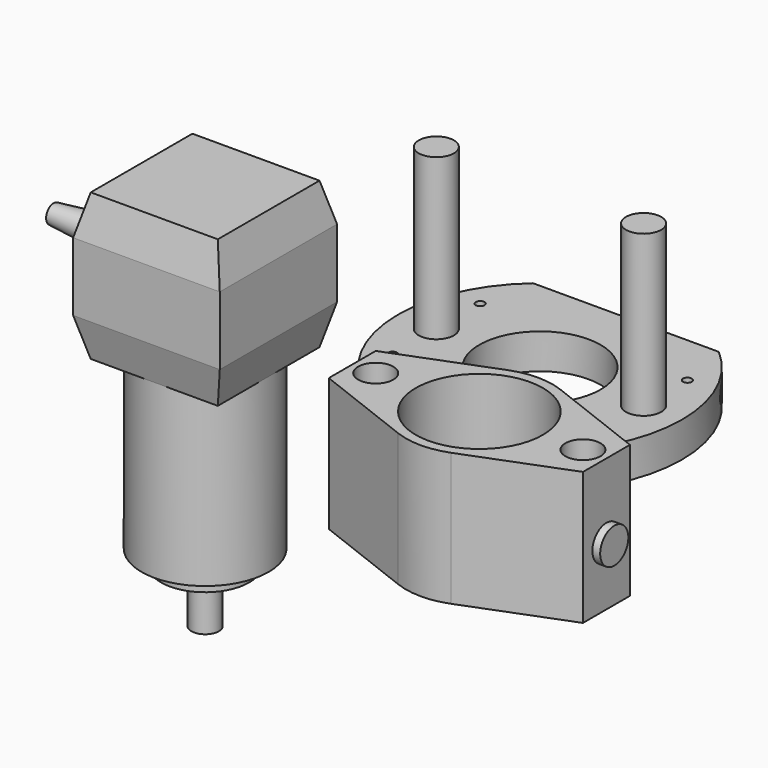
from build123d import *

# Parameters (mm, degrees)
F0_R         = 9
F0_R_2       = 31
F1_DEPTH     = 18
F2_DEPTH     = 100
F3_R         = 4.5
F4_DEPTH     = 100
F5_R         = 9
F5_R_2       = 32.5
F6_DEPTH     = 68
F7_R         = 9
F8_DEPTH     = 4
F9_R         = 9
F10_DEPTH    = 4
F16_W        = 75
F16_H        = 75
F17_DEPTH    = 75
F18_SIZE2    = 5
F18_SIZE     = 20
F19_C1_SIZE2 = 5
F19_C1_SIZE  = 20
F19_C2_SIZE2 = 5
F19_C2_SIZE  = 20
F19_C3_SIZE2 = 5
F19_C3_SIZE  = 20
F19_C4_SIZE2 = 20
F19_C4_SIZE  = 5
F19_C5_SIZE2 = 20
F19_C5_SIZE  = 5
F19_C6_SIZE2 = 5
F19_C6_SIZE  = 20
F19_C7_SIZE2 = 5
F19_C7_SIZE  = 20
F20_R        = 9
F21_DEPTH    = 40
F21_TAPER    = 6
F22_R        = 32.5
F23_DEPTH    = 88
F24_R        = 22.5
F25_DEPTH    = 8
F26_R        = 7
F27_DEPTH    = 27
F28_R        = 2.25
F29_DEPTH    = 25


# Not quite as in the source:
# - a feature of the source that left no trace in its solid (it failed there, or was rolled back) is left out


with BuildPart() as f1:
    # F0 (on Top) → F1 (new body)
    with BuildSketch(Plane.XY):
        with BuildLine():
            Line((47.5, 55), (-47.5, 55))
            ThreePointArc((-47.5, 55), (-72.6722092687, 0), (-47.5, -55))
            Line((-47.5, -55), (47.5, -55))
            ThreePointArc((47.5, -55), (72.6722092687, 0), (47.5, 55))
        make_face()
        with Locations((-53, 0)):
            Circle(F0_R, mode=Mode.SUBTRACT)
        Circle(F0_R_2, mode=Mode.SUBTRACT)
        with Locations((53, 0)):
            Circle(F0_R, mode=Mode.SUBTRACT)
    extrude(amount=F1_DEPTH)

    # F0 (on Top) → F2 (join)
    with BuildSketch(Plane.XY):
        with Locations((-53, 0)):
            Circle(F0_R)
        with Locations((53, 0)):
            Circle(F0_R)
    extrude(amount=F2_DEPTH)

    # F3 (on Right) → F4 (cut, symmetric)
    with BuildSketch(Plane.YZ):
        with Locations((-41.5, 9)):
            Circle(F3_R)
        with Locations((41.5, 9)):
            Circle(F3_R)
    extrude(amount=F4_DEPTH, both=True, mode=Mode.SUBTRACT)

    # F28 (on face) → F29 (cut)
    with BuildSketch(Plane.XY):
        with Locations((-53, 28)):
            Circle(F28_R)
        with Locations((-53, -28)):
            Circle(F28_R)
        with Locations((53, -28)):
            Circle(F28_R)
        with Locations((53, 28)):
            Circle(F28_R)
    extrude(amount=F29_DEPTH, mode=Mode.SUBTRACT)


with BuildPart() as f6:
    # F5 (on Top) → F6 (new body)
    with BuildSketch(Plane.XY):
        with BuildLine():
            Line((0, -105), (0, -135))
            Line((0, -135), (51.4330297899, -154.9597957562))
            ThreePointArc((51.4330297899, -154.9597957562), (65, -157.5), (78.5669702101, -154.9597957562))
            Line((78.5669702101, -154.9597957562), (130, -135))
            Line((130, -135), (130, -105))
            Line((130, -105), (78.5669702101, -85.0402042438))
            ThreePointArc((78.5669702101, -85.0402042438), (65, -82.5), (51.4330297899, -85.0402042438))
            Line((51.4330297899, -85.0402042438), (0, -105))
        make_face()
        with Locations((12, -120)):
            Circle(F5_R, mode=Mode.SUBTRACT)
        with Locations((65, -120)):
            Circle(F5_R_2, mode=Mode.SUBTRACT)
        with Locations((118, -120)):
            Circle(F5_R, mode=Mode.SUBTRACT)
    extrude(amount=F6_DEPTH)

    # F7 (on face) → F8 (join)
    with BuildSketch(Plane.YZ.offset(130)):
        with Locations((-120, 30)):
            Circle(F7_R)
    extrude(amount=F8_DEPTH)

    # F9 (on face) → F10 (join)
    with BuildSketch(Plane(origin=(0, 0, 0), x_dir=(0, -1, 0), z_dir=(-1, 0, 0))):
        with Locations((120, 30)):
            Circle(F9_R)
    extrude(amount=F10_DEPTH)


with BuildPart() as f17:
    # F16 (on Top) → F17 (new body)
    with BuildSketch(Plane.XY):
        with Locations((-133.6621306837, -46.9966906275)):
            Rectangle(F16_W, F16_H)
    extrude(amount=F17_DEPTH)

    # F18
    f18_edges = [f17.edges().sort_by_distance(p)[0] for p in [
        (-96.162131, -46.996691, 75),
    ]]
    f18_side = f17.faces().sort_by_distance((-96.162131, -46.996691, 37.5))[0]
    chamfer(f18_edges, length=F18_SIZE, length2=F18_SIZE2, reference=f18_side)

    # F19: chamfer of 20 x 5 on 7 edges, made by hand

    # F19_c1
    f19_c1_edges = [f17.edges().sort_by_distance(p)[0] for p in [
        (-133.6621306837, -9.4966906275, 0),
    ]]
    f19_c1_side = f17.faces().sort_by_distance((-133.6621306837, -9.4966906275, 0.1))[0]
    chamfer(f19_c1_edges, length=F19_C1_SIZE, length2=F19_C1_SIZE2, reference=f19_c1_side)

    # F19_c2
    f19_c2_edges = [f17.edges().sort_by_distance(p)[0] for p in [
        (-136.1621306837, -9.4966906275, 75),
    ]]
    f19_c2_side = f17.faces().sort_by_distance((-136.1621306837, -9.4966906275, 74.9))[0]
    chamfer(f19_c2_edges, length=F19_C2_SIZE, length2=F19_C2_SIZE2, reference=f19_c2_side)

    # F19_c3
    f19_c3_edges = [f17.edges().sort_by_distance(p)[0] for p in [
        (-96.1621306837, -49.4966906275, 0),
    ]]
    f19_c3_side = f17.faces().sort_by_distance((-96.1621306837, -49.4966906275, 0.1))[0]
    chamfer(f19_c3_edges, length=F19_C3_SIZE, length2=F19_C3_SIZE2, reference=f19_c3_side)

    # F19_c4
    f19_c4_edges = [f17.edges().sort_by_distance(p)[0] for p in [
        (-171.1621306837, -49.4966906275, 0),
    ]]
    f19_c4_side = f17.faces().sort_by_distance((-171.0621306837, -49.4966906275, 0))[0]
    chamfer(f19_c4_edges, length=F19_C4_SIZE, length2=F19_C4_SIZE2, reference=f19_c4_side)

    # F19_c5
    f19_c5_edges = [f17.edges().sort_by_distance(p)[0] for p in [
        (-133.6621306837, -84.4966906275, 0),
    ]]
    f19_c5_side = f17.faces().sort_by_distance((-133.6621306837, -84.3966906275, 0))[0]
    chamfer(f19_c5_edges, length=F19_C5_SIZE, length2=F19_C5_SIZE2, reference=f19_c5_side)

    # F19_c6
    f19_c6_edges = [f17.edges().sort_by_distance(p)[0] for p in [
        (-171.1621306837, -49.4966906275, 75),
    ]]
    f19_c6_side = f17.faces().sort_by_distance((-171.1621306837, -49.4966906275, 74.9))[0]
    chamfer(f19_c6_edges, length=F19_C6_SIZE, length2=F19_C6_SIZE2, reference=f19_c6_side)

    # F19_c7
    f19_c7_edges = [f17.edges().sort_by_distance(p)[0] for p in [
        (-133.6621306837, -84.4966906275, 75),
    ]]
    f19_c7_side = f17.faces().sort_by_distance((-133.6621306837, -84.4966906275, 74.9))[0]
    chamfer(f19_c7_edges, length=F19_C7_SIZE, length2=F19_C7_SIZE2, reference=f19_c7_side)

    # F20 (on face) → F21 (join)
    with BuildSketch(Plane(origin=(-171.1621306837, 0, 0), x_dir=(0, -1, 0), z_dir=(-1, 0, 0))):
        with Locations((46.9966906275, 37.5)):
            Circle(F20_R)
    extrude(amount=F21_DEPTH, taper=F21_TAPER)

    # F22 (on face) → F23 (join)
    with BuildSketch(Plane(origin=(0, 0, 0), x_dir=(1, 0, 0), z_dir=(0, 0, -1))):
        with Locations((-133.6621306837, 46.9966906275)):
            Circle(F22_R)
    extrude(amount=F23_DEPTH)

    # F24 (on face) → F25 (join)
    with BuildSketch(Plane(origin=(0, 0, -88), x_dir=(1, 0, 0), z_dir=(0, 0, -1))):
        with Locations((-133.6621306837, 46.9966906275)):
            Circle(F24_R)
    extrude(amount=F25_DEPTH)

    # F26 (on face) → F27 (join)
    with BuildSketch(Plane(origin=(0, 0, -96), x_dir=(1, 0, 0), z_dir=(0, 0, -1))):
        with Locations((-133.6621306837, 46.9966906275)):
            Circle(F26_R)
    extrude(amount=F27_DEPTH)


solid = Compound([f1.part, f6.part, f17.part])
